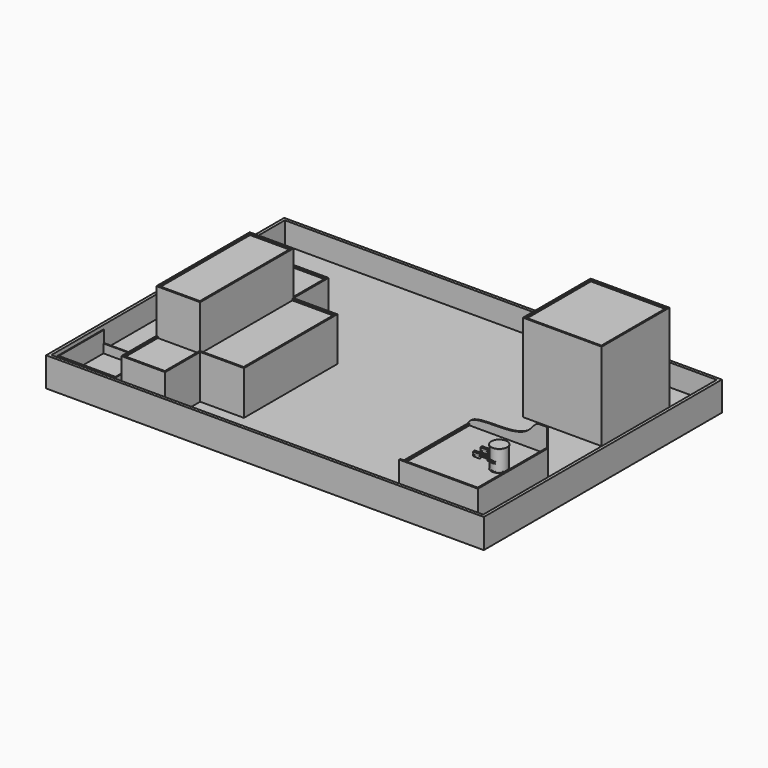
from build123d import *

# Parameters (mm, degrees)
F0_R      = 27.2
F1_DEPTH  = 2.83
F2_R      = 26.4
F3_DEPTH  = 67.36
F4_R      = 27.2
F5_DEPTH  = 2.83
F9_W      = 270
F9_H      = 300
F10_DEPTH = 72
F12_DEPTH = 15
F14_DEPTH = 5
F15_W     = 5
F15_H     = 290
F16_DEPTH = 5
F17_W     = 1500
F17_H     = 1020
F18_DEPTH = 25
F19_W     = 270
F19_H     = 290
F20_DEPTH = 300
F21_W     = 260
F21_H     = 280
F22_DEPTH = 5
F23_W     = 1500
F23_H     = 1020
F23_W_2   = 1480
F23_H_2   = 1000
F24_DEPTH = 75
F26_DEPTH = 150
F27_W     = 150
F27_H     = 400
F28_DEPTH = 150
F29_W     = 140
F29_H     = 390
F30_DEPTH = 5
F31_W     = 140
F31_H     = 145
F31_W_2   = 145
F31_H_2   = 390
F32_DEPTH = 5
F33_R     = 3
F34_DEPTH = 4
F35_R     = 3.99999
F35_2_R   = 3.99999
F36_R     = 3
F37_DEPTH = 8
F38_R     = 3
F39_DEPTH = 8
F40_R     = 3
F40_R_2   = 2.5
F41_DEPTH = 3
F42_R     = 3
F42_R_2   = 2.5
F43_DEPTH = 3
F45_DEPTH = 270.001
F46_W     = 200
F46_H     = 200
F46_W_2   = 194
F46_H_2   = 191
F47_DEPTH = 30
F49_DEPTH = 40
F50_R     = 2.5
F51_DEPTH = 8
F53_R     = 3
F54_DEPTH = 6


# Not quite as in the source:
# - a fillet or chamfer is up to 0.001 mm smaller than in the source, because OpenCascade refuses the exact size
# - a feature names something its author has since deleted; it is built from what else it names


with BuildPart() as f1:
    # F0 (on Top) → F1 (new body)
    with BuildSketch(Plane.XY):
        Circle(F0_R)
    extrude(amount=F1_DEPTH)

    # F2 (on face) → F3 (join)
    with BuildSketch(Plane.XY.offset(2.83)):
        Circle(F2_R)
    extrude(amount=F3_DEPTH)

    # F4 (on face) → F5 (join)
    with BuildSketch(Plane.XY.offset(70.19)):
        Circle(F4_R)
    extrude(amount=F5_DEPTH)


with BuildPart() as f10:
    # F9 (on Top) → F10 (new body)
    with BuildSketch(Plane.XY):
        with Locations((-87.8, 0)):
            Rectangle(F9_W, F9_H)
    extrude(amount=-F10_DEPTH)

    # F11 (on face) → F12 (join)
    with BuildSketch(Plane.XY):
        Polygon((-222.8, -145), (-222.8, -150), (47.2, -150), (47.2, 150), (42.2, 150), (42.2, -145), align=None)
    extrude(amount=F12_DEPTH)

    # F13 (on face) → F14 (join)
    with BuildSketch(Plane(origin=(0, 150, 0), x_dir=(-1, 0, 0), z_dir=(0, 1, 0))):
        with BuildLine():
            Line((-21.3134280931, 81.3575685024), (-47.2, 81.3575685024))
            Line((-47.2, 81.3575685024), (-47.2, -72))
            Line((-47.2, -72), (222.8, -72))
            Line((222.8, -72), (222.8, 0))
            add(Edge.make_bspline(
                [(-21.3134280931, 81.3575685024), (-6.3059147253, 81.3822787863), (12.9585432644, 38.1268753575), (103.6097013063, 23.6068887567), (223.0224295336, 30.7718731823), (222.8, 0)],
                knots=[0, 0, 0, 0, 0.2487100673, 0.6151112321, 1, 1, 1, 1], degree=3))
        make_face()
    extrude(amount=-F14_DEPTH)

    # F15 (on face) → F16 (join)
    with BuildSketch(Plane.XY):
        with Locations((-220.3, 0)):
            Rectangle(F15_W, F15_H)
    extrude(amount=F16_DEPTH)

    # F17 (on face) → F18 (join)
    with BuildSketch(Plane(origin=(0, 0, -72), x_dir=(1, 0, 0), z_dir=(0, 0, -1))):
        with Locations((-602.8, -260)):
            Rectangle(F17_W, F17_H)
    extrude(amount=F18_DEPTH)

    # F19 (on face) → F20 (join)
    with BuildSketch(Plane.XY.offset(-72)):
        with Locations((-87.8, 525)):
            Rectangle(F19_W, F19_H)
    extrude(amount=F20_DEPTH)

    # F21 (on face) → F22 (cut)
    with BuildSketch(Plane.XY.offset(228)):
        with Locations((-87.8, 525)):
            Rectangle(F21_W, F21_H)
    extrude(amount=-F22_DEPTH, mode=Mode.SUBTRACT)

    # F23 (on face) → F24 (join)
    with BuildSketch(Plane.XY.offset(-72)):
        with Locations((-602.8, 260)):
            Rectangle(F23_W, F23_H)
        with Locations((-602.8, 260)):
            Rectangle(F23_W_2, F23_H_2, mode=Mode.SUBTRACT)
    extrude(amount=F24_DEPTH)

    # F25 (on face) → F26 (join)
    with BuildSketch(Plane.XY.offset(-72)):
        Polygon((-952.8, 460), (-1102.8, 460), (-1102.8, -240), (-952.8, -240), (-952.8, -90), (-802.8, -90), (-802.8, 310), (-952.8, 310), align=None)
    extrude(amount=F26_DEPTH)

    # F27 (on face) → F28 (join)
    with BuildSketch(Plane.XY.offset(78)):
        with Locations((-1027.8, 110)):
            Rectangle(F27_W, F27_H)
    extrude(amount=F28_DEPTH)

    # F29 (on face) → F30 (cut)
    with BuildSketch(Plane.XY.offset(228)):
        with Locations((-1027.8, 110)):
            Rectangle(F29_W, F29_H)
    extrude(amount=-F30_DEPTH, mode=Mode.SUBTRACT)

    # F31 (on face) → F32 (cut)
    with BuildSketch(Plane.XY.offset(78)):
        with Locations((-1027.8, 382.5)):
            Rectangle(F31_W, F31_H)
        with Locations((-880.3, 110)):
            Rectangle(F31_W_2, F31_H_2)
        with Locations((-1027.8, -162.5)):
            Rectangle(F31_W, F31_H)
    extrude(amount=-F32_DEPTH, mode=Mode.SUBTRACT)

    # F46 (on face) → F47 (join)
    with BuildSketch(Plane.XY.offset(-72)):
        with Locations((-1232.8, -130)):
            Rectangle(F46_W, F46_H)
        with Locations((-1232.8, -128.5)):
            Rectangle(F46_W_2, F46_H_2, mode=Mode.SUBTRACT)
    extrude(amount=F47_DEPTH)

    # F48 (on face) → F49 (join)
    with BuildSketch(Plane.XY.offset(-42)):
        Polygon((-1329.8, -30), (-1332.8, -30), (-1332.8, -230), (-1329.8, -230), (-1135.8, -230), (-1132.8, -230), (-1132.8, -30), (-1135.8, -30), (-1135.8, -224), (-1329.8, -224), align=None)
    extrude(amount=F49_DEPTH)


with BuildPart() as f34:
    # F33 (on offset) → F34 (new body, symmetric)
    with BuildSketch(Plane.XY.offset(25)):
        with BuildLine():
            Line((-55, -12), (-74.5, -12))
            Line((-74.5, -12), (-74.5, -13))
            Line((-74.5, -13), (-65.6457513111, -13))
            ThreePointArc((-65.6457513111, -13), (-67, -16), (-65.6457513111, -19))
            Line((-65.6457513111, -19), (-74.5, -19))
            Line((-74.5, -19), (-74.5, -20))
            Line((-74.5, -20), (-55, -20))
            ThreePointArc((-55, -20), (-51, -16), (-55, -12))
        make_face()
        with Locations((-63, -16)):
            Circle(F33_R, mode=Mode.SUBTRACT)
        with Locations((-55, -16)):
            Circle(F33_R, mode=Mode.SUBTRACT)
    extrude(amount=F34_DEPTH, both=True)

    # F35 (radius 4 in the source; OpenCascade refuses exactly that, so slightly less here)
    f35_edges = [f34.edges().sort_by_distance(p)[0] for p in [
        (-74.5, -19.5, 29),
        (-74.5, -12.5, 29),
        (-74.5, -19.5, 21),
        (-74.5, -12.5, 21),
    ]]
    fillet(f35_edges, radius=F35_R)

    # F36 (on face) → F37 (join, through all)
    with BuildSketch(Plane.XZ.offset(20)):
        with Locations((-70.5, 25)):
            Circle(F36_R)
    extrude(amount=-F37_DEPTH)

    # F42 (on offset) → F43 (join, symmetric)
    with BuildSketch(Plane.XY.offset(25)):
        with Locations((-63, -16)):
            Circle(F42_R)
        with Locations((-63, -16)):
            Circle(F42_R_2, mode=Mode.SUBTRACT)
        with Locations((-55, -16)):
            Circle(F42_R)
        with Locations((-55, -16)):
            Circle(F42_R_2, mode=Mode.SUBTRACT)
    extrude(amount=F43_DEPTH, both=True)


with BuildPart() as f34b:
    # F33 (on offset) → F34, piece 2 (new body, symmetric)
    with BuildSketch(Plane.XY.offset(25)):
        with BuildLine():
            Line((-74.5, 13), (-74.5, 12))
            Line((-74.5, 12), (-55, 12))
            ThreePointArc((-55, 12), (-51, 16), (-55, 20))
            Line((-55, 20), (-74.5, 20))
            Line((-74.5, 20), (-74.5, 19))
            Line((-74.5, 19), (-65.6457513111, 19))
            ThreePointArc((-65.6457513111, 19), (-67, 16), (-65.6457513111, 13))
            Line((-65.6457513111, 13), (-74.5, 13))
        make_face()
        with Locations((-63, 16)):
            Circle(F33_R, mode=Mode.SUBTRACT)
        with Locations((-55, 16)):
            Circle(F33_R, mode=Mode.SUBTRACT)
    extrude(amount=F34_DEPTH, both=True)

    # F35#2 (radius 4 in the source; OpenCascade refuses exactly that, so slightly less here)
    f35_2_edges = [f34b.edges().sort_by_distance(p)[0] for p in [
        (-74.5, 12.5, 29),
        (-74.5, 19.5, 29),
        (-74.5, 19.5, 21),
        (-74.5, 12.5, 21),
    ]]
    fillet(f35_2_edges, radius=F35_2_R)

    # F38 (on face) → F39 (join, through all)
    with BuildSketch(Plane(origin=(0, 20, 0), x_dir=(-1, 0, 0), z_dir=(0, 1, 0))):
        with Locations((70.5, 25)):
            Circle(F38_R)
    extrude(amount=-F39_DEPTH)

    # F40 (on offset) → F41 (join, symmetric)
    with BuildSketch(Plane.XY.offset(25)):
        with Locations((-55, 16)):
            Circle(F40_R)
        with Locations((-55, 16)):
            Circle(F40_R_2, mode=Mode.SUBTRACT)
        with Locations((-63, 16)):
            Circle(F40_R)
        with Locations((-63, 16)):
            Circle(F40_R_2, mode=Mode.SUBTRACT)
    extrude(amount=F41_DEPTH, both=True)


with BuildPart() as f45_tool:
    # F44 (on face) → F45 (new body, through all)
    with BuildSketch(Plane(origin=(0, 20, 0), x_dir=(-1, 0, 0), z_dir=(0, 1, 0))):
        with BuildLine():
            Line((71.5, 26), (71.5, 27.2912878475))
            ThreePointArc((71.5, 27.2912878475), (70.5, 27.5), (69.5, 27.2912878475))
            Line((69.5, 27.2912878475), (69.5, 26))
            Line((69.5, 26), (68.2087121525, 26))
            ThreePointArc((68.2087121525, 26), (68, 25), (68.2087121525, 24))
            Line((68.2087121525, 24), (69.5, 24))
            Line((69.5, 24), (69.5, 22.7087121525))
            ThreePointArc((69.5, 22.7087121525), (70.5, 22.5), (71.5, 22.7087121525))
            Line((71.5, 22.7087121525), (71.5, 24))
            Line((71.5, 24), (72.7912878475, 24))
            ThreePointArc((72.7912878475, 24), (73, 25), (72.7912878475, 26))
            Line((72.7912878475, 26), (71.5, 26))
        make_face()
    extrude(amount=-F45_DEPTH)


with BuildPart() as f34_1:
    add(f34.part)

    # F45: cut by f45_tool
    add(f45_tool.part, mode=Mode.SUBTRACT)


with BuildPart() as f34b_1:
    add(f34b.part)

    # F45: cut by f45_tool
    add(f45_tool.part, mode=Mode.SUBTRACT)


with BuildPart() as f51:
    # F50 (on face) → F51 (new body)
    with BuildSketch(Plane.XY.offset(29)):
        Polygon((-0.619225204, 27.0833074003), (-78.9677798748, 27.0833074003), (-78.9677798748, 12), (-44.8230803013, 12), (-44.8230803013, -8.2436139807), (-78.9677798748, -8.2436139807), (-78.9677798748, -29.8999884278), (-0.619225204, -29.8999884278), align=None)
        with Locations((-63, 16)):
            Circle(F50_R, mode=Mode.SUBTRACT)
    extrude(amount=F51_DEPTH)


with BuildPart() as f54:
    # F53 (on face) → F54 (new body)
    with BuildSketch(Plane.XY.offset(29)):
        Polygon((-27.5974007475, 19.9976182654), (-74.2540242302, 19.9976182654), (-74.2540242302, 11.6435588449), (-30.884288795, 11.6435588449), (-30.884288795, 4.3928670809), (-30.884288795, -2.5425766483), (-30.884288795, -7.5865354277), (-30.884288795, -12), (-74.2540242302, -12), (-74.2540242302, -20.0388085917), (-26.6516575741, -20.0388085917), (-16.0766760039, -28.607969068), (-6.900405899, -30.9904933795), (5.3059876971, -30.9904933795), (10.81732286, -28.425222185), (3.7697205168, -28.9575885981), (-15.0486715138, -24.8369798064), (-27.4104960263, -12.6399816945), (-27.4104960263, 11.9188399985), (-23.125063628, 18.3469895273), (-16.037620604, 24.6103126556), (3.7697205168, 29.6126633063), (-0.8013676654, 31.3465270326), (-10.4164149764, 30.0855330303), (-20.189083569, 27.0906846151), align=None)
        with Locations((-63, -16)):
            Circle(F53_R, mode=Mode.SUBTRACT)
        with Locations((-55, -16)):
            Circle(F53_R, mode=Mode.SUBTRACT)
        with Locations((-63, 16)):
            Circle(F53_R, mode=Mode.SUBTRACT)
        with Locations((-55, 16)):
            Circle(F53_R, mode=Mode.SUBTRACT)
    extrude(amount=F54_DEPTH)


solid = Compound([f1.part, f10.part, f34_1.part, f34b_1.part, f54.part])
